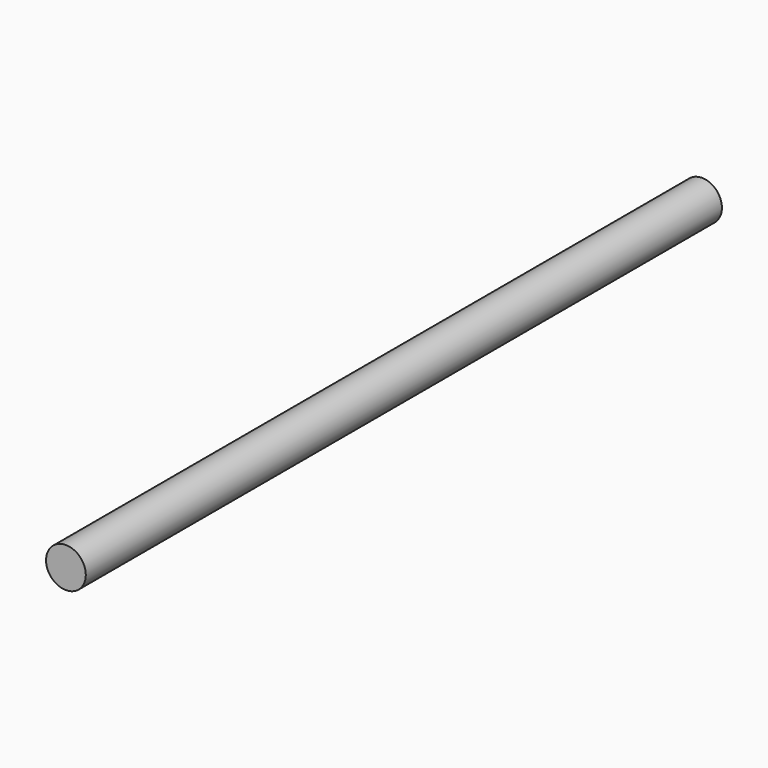
from build123d import *

# Parameters (mm, degrees)
F0_R     = 3.175
F1_DEPTH = 127


# Not quite as in the source:
# - the program builds the solid bodies; features that only make, move or delete a surface that nothing else refers to are left out


with BuildPart() as f1:
    # F0 (on Front) → F1 (new body)
    with BuildSketch(Plane.XZ):
        with Locations((-40.2976833284, 34.791637212)):
            Circle(F0_R)
    extrude(amount=F1_DEPTH)


solid = f1.part
